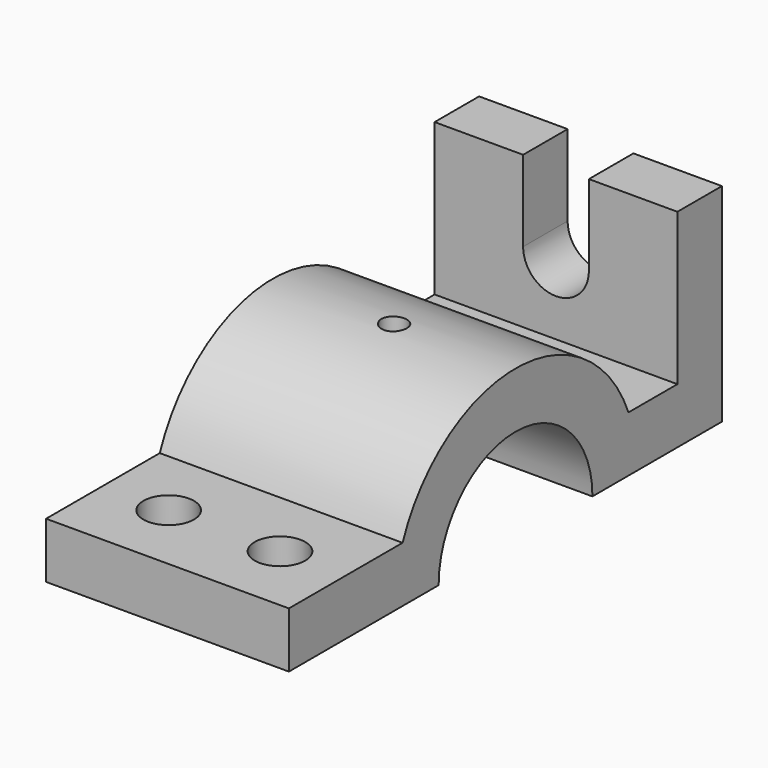
from build123d import *

# Parameters (mm, degrees)
F0_W     = 11
F0_H     = 30
F1_DEPTH = 24
F3_DEPTH = 17.9
F4_R     = 5
F4_R_2   = 2.5
F5_DEPTH = 51.2


with BuildPart() as f1:
    # F0 (on Right) → F1 (new body, symmetric)
    with BuildSketch(Plane.YZ):
        with BuildLine():
            Line((-56, 0), (-30, 0))
            ThreePointArc((-30, 0), (-29.4730143031, 5.5983415304), (-27.9105714739, 11))
            Line((-27.9105714739, 11), (-56, 11))
            Line((-56, 11), (-56, 0))
        make_face()
        with BuildLine():
            ThreePointArc((-27.9105714739, 11), (-29.4730143031, 5.5983415304), (-30, 0))
            Line((-30, 0), (-19, 0))
            ThreePointArc((-19, 0), (-18.1017503893, 5.7729223833), (-15.4919333848, 11))
            Line((-15.4919333848, 11), (-27.9105714739, 11))
        make_face()
        with BuildLine():
            Line((15.4919333848, 11), (27.9105714739, 11))
            ThreePointArc((27.9105714739, 11), (0, 30), (-27.9105714739, 11))
            Line((-27.9105714739, 11), (-15.4919333848, 11))
            ThreePointArc((-15.4919333848, 11), (0, 19), (15.4919333848, 11))
        make_face()
        with BuildLine():
            Line((19, 0), (30, 0))
            ThreePointArc((30, 0), (29.4730143031, 5.5983415304), (27.9105714739, 11))
            Line((27.9105714739, 11), (15.4919333848, 11))
            ThreePointArc((15.4919333848, 11), (18.1017503893, 5.7729223833), (19, 0))
        make_face()
        with BuildLine():
            ThreePointArc((27.9105714739, 11), (29.4730143031, 5.5983415304), (30, 0))
            Line((30, 0), (51, 0))
            Line((51, 0), (51, 11))
            Line((51, 11), (40, 11))
            Line((40, 11), (27.9105714739, 11))
        make_face()
        with Locations((45.5, 26)):
            Rectangle(F0_W, F0_H)
    extrude(amount=F1_DEPTH, both=True)

    # F2 (on face) → F3 (cut, symmetric)
    with BuildSketch(Plane(origin=(0, 51, 0), x_dir=(-1, 0, 0), z_dir=(0, 1, 0))):
        with BuildLine():
            ThreePointArc((-6.5, 25), (0, 18.5), (6.5, 25))
            ThreePointArc((6.5, 25), (0, 31.5), (-6.5, 25))
        make_face()
        with BuildLine():
            ThreePointArc((-6.5, 25), (0, 31.5), (6.5, 25))
            Line((6.5, 25), (6.5, 41))
            Line((6.5, 41), (-6.5, 41))
            Line((-6.5, 41), (-6.5, 25))
        make_face()
    extrude(amount=F3_DEPTH, both=True, mode=Mode.SUBTRACT)

    # F4 (on Top) → F5 (cut, symmetric)
    with BuildSketch(Plane.XY):
        with Locations((-11, -41.955285737)):
            Circle(F4_R)
        with Locations((11, -41.955285737)):
            Circle(F4_R)
        Circle(F4_R_2)
    extrude(amount=F5_DEPTH, both=True, mode=Mode.SUBTRACT)


solid = f1.part
